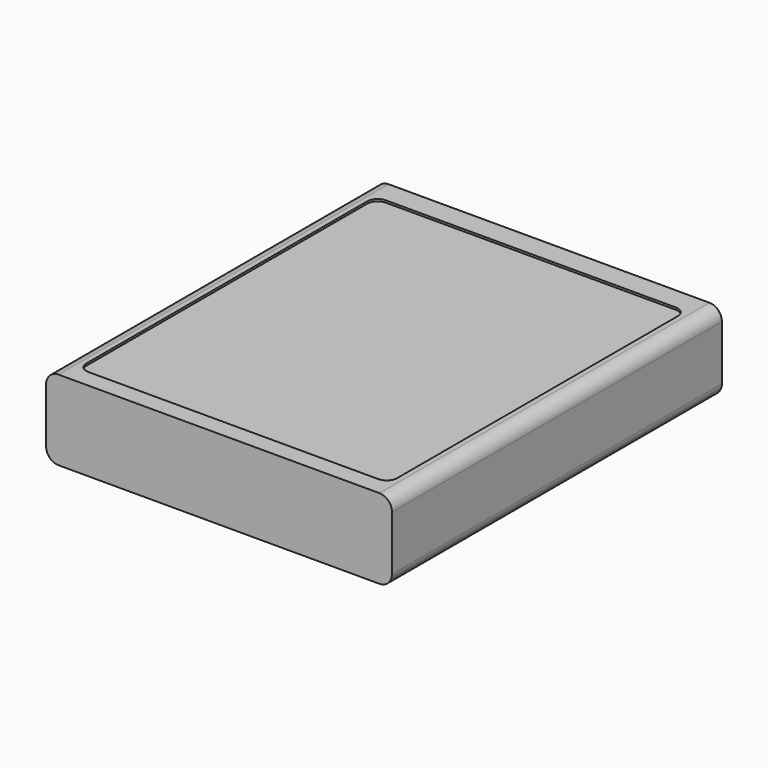
from build123d import *

# Parameters (mm, degrees)
F0_W      = 82.55
F0_H      = 98.425
F2_DEPTH  = 19.05
F3_R      = 3
F4_W      = 76.55
F4_H      = 13.05
F5_DEPTH  = 6.35
F6_W      = 36.55
F6_H      = 2.2
F7_DEPTH  = 2
F8_W      = 8.7
F8_H      = 2.2
F9_DEPTH  = 25
F10_W     = 6
F10_H     = 2.2
F11_DEPTH = 6.35
F12_SIZE  = 1.09999
F14_DEPTH = 0.5


# Not quite as in the source:
# - a fillet or chamfer is up to 0.001 mm smaller than in the source, because OpenCascade refuses the exact size


with BuildPart() as f2:
    # F0 (on Top) → F2 (new body)
    with BuildSketch(Plane.XY):
        with Locations((-41.275, 49.2125)):
            Rectangle(F0_W, F0_H)
    extrude(amount=-F2_DEPTH)

    # F3
    f3_edges = [f2.edges().sort_by_distance(p)[0] for p in [
        (-82.55, 49.2125, -19.05),
        (-82.55, 49.2125, 0),
        (0, 49.2125, 0),
        (0, 49.2125, -19.05),
    ]]
    fillet(f3_edges, radius=F3_R)

    # F4 (on face) → F5 (cut)
    with BuildSketch(Plane(origin=(0, 98.425, 0), x_dir=(-1, 0, 0), z_dir=(0, 1, 0))):
        with Locations((41.275, -9.525)):
            Rectangle(F4_W, F4_H)
    extrude(amount=-F5_DEPTH, mode=Mode.SUBTRACT)

    # F6 (on face) → F7 (cut)
    with BuildSketch(Plane(origin=(0, 92.075, 0), x_dir=(-1, 0, 0), z_dir=(0, 1, 0))):
        with Locations((41.275, -9.55)):
            Rectangle(F6_W, F6_H)
    extrude(amount=-F7_DEPTH, mode=Mode.SUBTRACT)

    # F8 (on face) → F9 (cut)
    with BuildSketch(Plane(origin=(0, 92.075, 0), x_dir=(-1, 0, 0), z_dir=(0, 1, 0))):
        with Locations((66.3, -9.55)):
            Rectangle(F8_W, F8_H)
        with Locations((16.25, -9.55)):
            Rectangle(F8_W, F8_H)
    extrude(amount=-F9_DEPTH, mode=Mode.SUBTRACT)

    # F10 (on face) → F11 (join, through all)
    with BuildSketch(Plane(origin=(0, 92.075, 0), x_dir=(-1, 0, 0), z_dir=(0, 1, 0))):
        with Locations((73.65, -9.55)):
            Rectangle(F10_W, F10_H)
        with Locations((8.9, -9.55)):
            Rectangle(F10_W, F10_H)
    extrude(amount=F11_DEPTH)

    # F12 (size 1.1 in the source; OpenCascade refuses exactly that, so slightly less here)
    f12_edges = [f2.edges().sort_by_distance(p)[0] for p in [
        (-8.9, 98.425, -8.45),
        (-8.9, 98.425, -10.65),
        (-73.65, 98.425, -8.45),
        (-73.65, 98.425, -10.65),
    ]]
    chamfer(f12_edges, length=F12_SIZE)

    # F13 (on face) → F14 (cut)
    with BuildSketch(Plane.XY):
        with BuildLine():
            Line((-6.7, 93.025), (-75.85, 93.025))
            ThreePointArc((-75.85, 93.025), (-77.617766953, 92.292766953), (-78.35, 90.525))
            Line((-78.35, 90.525), (-78.35, 6.8))
            ThreePointArc((-78.35, 6.8), (-77.617766953, 5.032233047), (-75.85, 4.3))
            Line((-75.85, 4.3), (-6.7, 4.3))
            ThreePointArc((-6.7, 4.3), (-4.932233047, 5.032233047), (-4.2, 6.8))
            Line((-4.2, 6.8), (-4.2, 90.525))
            ThreePointArc((-4.2, 90.525), (-4.932233047, 92.292766953), (-6.7, 93.025))
        make_face()
    extrude(amount=-F14_DEPTH, mode=Mode.SUBTRACT)


solid = f2.part
